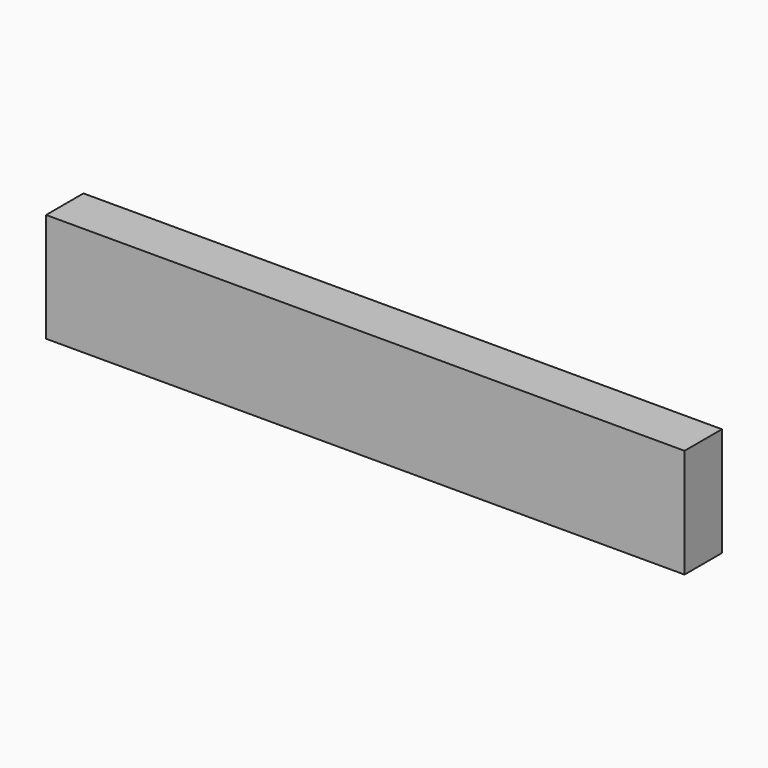
from build123d import *

# Parameters (mm, degrees)
F0_W     = 38.1
F0_H     = 88.9
F1_DEPTH = 260.35


with BuildPart() as f1:
    # F0 (on Right) → F1 (new body, symmetric)
    with BuildSketch(Plane.YZ):
        Rectangle(F0_W, F0_H)
    extrude(amount=F1_DEPTH, both=True)


solid = f1.part
